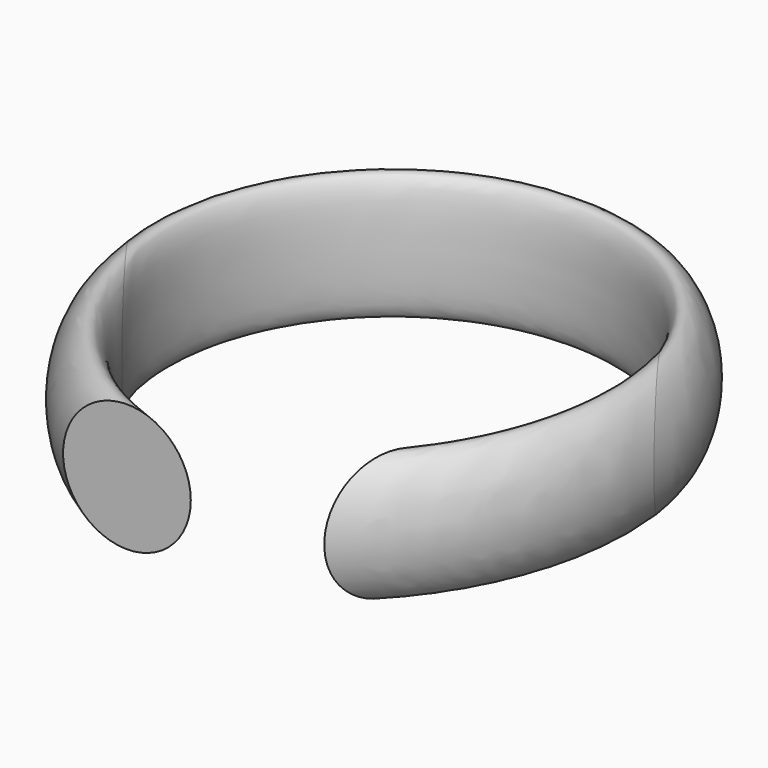
from build123d import *

# Parameters (mm, degrees)
F1_R = 12.506492


with BuildPart() as f2:
    # F2: sweep along a path in F0
    with BuildLine(Plane.XY) as f2_path:
        ThreePointArc((24.563487, 5.595358), (41.085497, 25.675696), (47.001004, 50.997693))
        ThreePointArc((47.001004, 50.997693), (2.717745, 95.280953), (-41.565515, 50.997693))
        ThreePointArc((-41.565515, 50.997693), (-35.388654, 25.472425), (-18.22488, 5.595358))
    # F1 (on Front) → F2 (sweep)
    with BuildSketch(Plane.XZ):
        with Locations((-8.454271, 0)):
            Circle(F1_R)
    sweep(path=f2_path.line)


solid = f2.part
